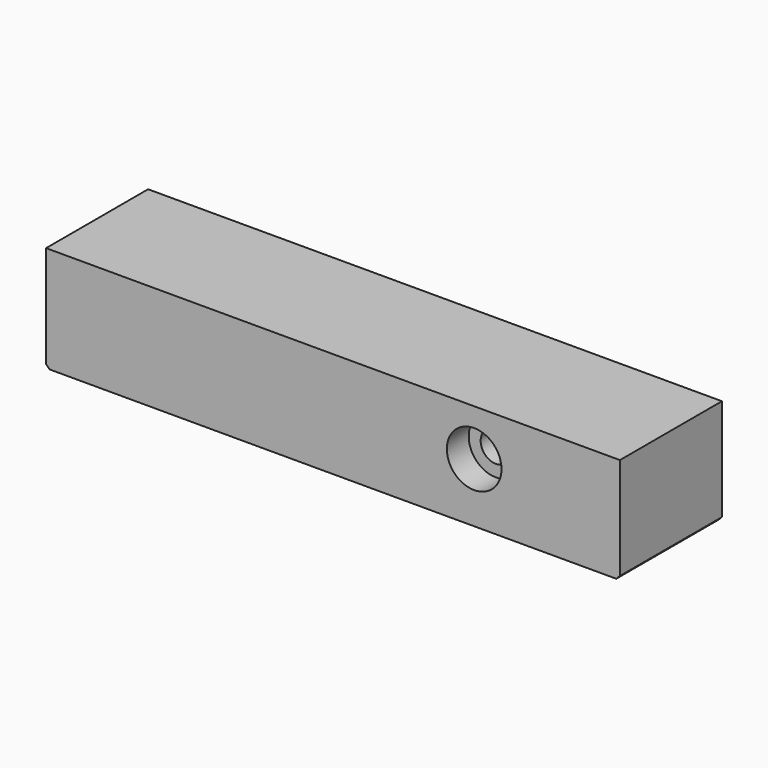
from build123d import *

# Parameters (mm, degrees)
F0_W      = 200.025
F0_H      = 76.2
F1_DEPTH  = 36.83
F2_DEPTH  = 31.75
F4_D      = 10.71626
F4_DEPTH  = 15.875
F4_TIP    = 3.2194893086
F5_D      = 12.7
F5_DEPTH  = 12.7
F5_TIP    = 3.8154649308
F6_SIZE   = 1.27
F7_R      = 9.525
F8_DEPTH  = 9.525
F10_D     = 10.71626
F10_DEPTH = 12.7
F10_TIP   = 3.2194893086


# Not quite as in the source:
# - a length typed as a fraction of an inch, garbled in the dataset ("3 / 203.2 mm" for 3/8 in), is restored
# - a feature names something its author has since deleted; it is built from what else it names


with BuildPart() as f1:
    # F0 (on Top) → F1 (new body)
    with BuildSketch(Plane.XY):
        with Locations((-0.1895949244, 0.1812406208)):
            Rectangle(F0_W, F0_H)
    extrude(amount=F1_DEPTH)

    # F2 (cut): a face of the model
    f2_faces = [f1.faces().sort_by_distance(p)[0] for p in [
        (-0.1895949244, 38.2812406208, 18.415),
    ]]
    extrude(f2_faces, amount=-F2_DEPTH, mode=Mode.SUBTRACT)

    # F4
    with Locations(Plane(origin=(0, 6.5312406208, 0), x_dir=(-1, 0, 0), z_dir=(0, 1, 0))):
        with Locations((-80.7729050756, 20.6248), (81.1520949244, 20.6248)):
            Hole(F4_D / 2, depth=F4_DEPTH)
            with Locations((0, 0, -(F4_DEPTH + F4_TIP / 2))):  # 118° drill point
                Cone(0, F4_D / 2, F4_TIP, mode=Mode.SUBTRACT)

    # F5
    with Locations(Plane(origin=(0, 6.5312406208, 0), x_dir=(-1, 0, 0), z_dir=(0, 1, 0))):
        with Locations((-49.0229050756, 20.6248), (49.4020949244, 20.6248)):
            Hole(F5_D / 2, depth=F5_DEPTH)
            with Locations((0, 0, -(F5_DEPTH + F5_TIP / 2))):  # 118° drill point
                Cone(0, F5_D / 2, F5_TIP, mode=Mode.SUBTRACT)

    # F6
    f6_edges = [f1.edges().sort_by_distance(p)[0] for p in [
        (-100.202095, -15.693759, 0),
        (99.822905, -15.693759, 0),
    ]]
    chamfer(f6_edges, length=F6_SIZE)

    # F7 (on face) → F8 (cut)
    with BuildSketch(Plane.XZ.offset(37.9187593792)):
        with Locations((49.0229050756, 20.6248)):
            Circle(F7_R)
    extrude(amount=-F8_DEPTH, mode=Mode.SUBTRACT)

    # F10
    with Locations(Plane.XZ.offset(28.3937593792)):
        with Locations((49.0229050756, 20.6248)):
            Hole(F10_D / 2, depth=F10_DEPTH)
            with Locations((0, 0, -(F10_DEPTH + F10_TIP / 2))):  # 118° drill point
                Cone(0, F10_D / 2, F10_TIP, mode=Mode.SUBTRACT)


solid = f1.part
